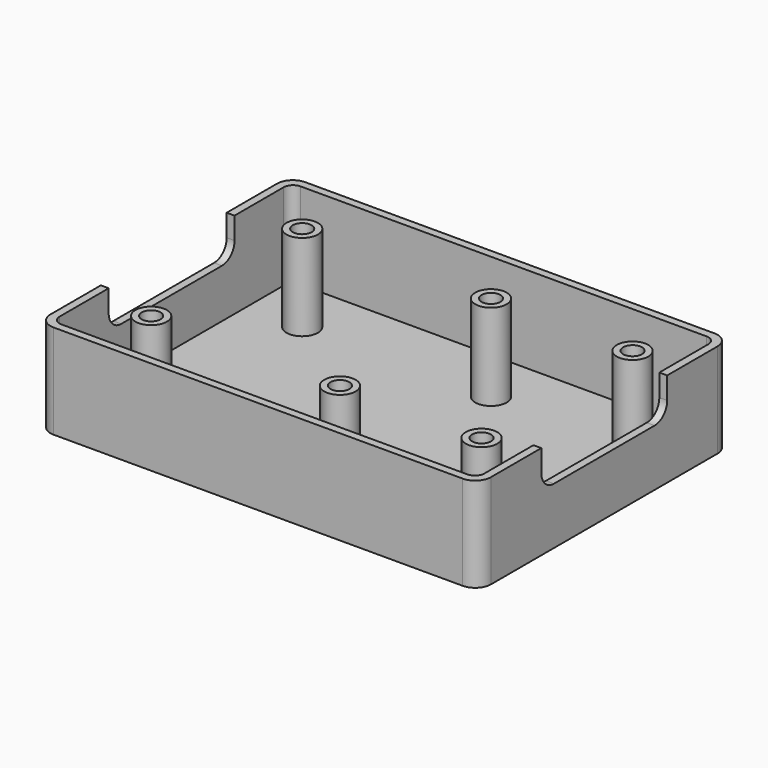
from build123d import *

# Parameters (mm, degrees)
F0_W          = 140
F0_H          = 100
F1_DEPTH      = 30
F2_T          = -2.5
F3_W          = 50
F3_H          = 12
F4_DEPTH      = 205.5
F5_R          = 5
F6_R          = 5
F7_R          = 3
F8_R          = 5
F9_DEPTH      = 27.5
F10_T         = 2
F10_T3_DEPTH  = 93
F10_T5_DEPTH  = 133
F10_T8_ANGLE  = 90.000000001
F10_T10_ANGLE = 90.000000001
F10_T12_ANGLE = 90.000000001
F10_T14_ANGLE = 90.000000001
F11_ANGLE     = 60
F12_ANGLE     = 30
F13_ANGLE     = 90


# Not quite as in the source:
# - a shell that OpenCascade refuses in one call is made with other operations: the cavity is built on its own and cut out


with BuildPart() as f1:
    # F0 (on Top) → F1 (new body)
    with BuildSketch(Plane.XY):
        with Locations((50, 0)):
            Rectangle(F0_W, F0_H)
    extrude(amount=F1_DEPTH)

    # F2
    f2_openings = [f1.faces().sort_by_distance(p)[0] for p in [
        (50, 0, 30),
    ]]
    offset(amount=F2_T, openings=f2_openings)

    # F3 (on face) → F4 (cut)
    with BuildSketch(Plane.YZ.offset(120)):
        with Locations((0, 24)):
            Rectangle(F3_W, F3_H)
    extrude(amount=-F4_DEPTH, mode=Mode.SUBTRACT)

    # F5
    f5_edges = [f1.edges().sort_by_distance(p)[0] for p in [
        (-18.75, 25, 18),
        (-18.75, -25, 18),
        (118.75, -25, 18),
        (118.75, 25, 18),
    ]]
    fillet(f5_edges, radius=F5_R)

    # F6
    f6_edges = [f1.edges().sort_by_distance(p)[0] for p in [
        (120, 50, 15),
        (-20, 50, 15),
        (-20, -50, 15),
        (120, -50, 15),
    ]]
    fillet(f6_edges, radius=F6_R)

    # F7
    f7_edges = [f1.edges().sort_by_distance(p)[0] for p in [
        (-17.5, -47.5, 16.25),
        (-17.5, 47.5, 16.25),
        (117.5, 47.5, 16.25),
        (117.5, -47.5, 16.25),
    ]]
    fillet(f7_edges, radius=F7_R)

    # F8 (on face) → F9 (join, through all)
    with BuildSketch(Plane.XY.offset(2.5)):
        with Locations((-5, -30)):
            Circle(F8_R)
        with Locations((40, -30)):
            Circle(F8_R)
        with Locations((100, -30)):
            Circle(F8_R)
        with Locations((100, 30)):
            Circle(F8_R)
        with Locations((40, 30)):
            Circle(F8_R)
        with Locations((-5, 30)):
            Circle(F8_R)
    extrude(amount=F9_DEPTH)

    # F10: shell of thickness 2, made by hand


with BuildPart() as f10_core1:
    # F10_t2: copy of F1
    add(f1.part)

    # the walls: a layer under each face that stays
    f10_faces = [f10_core1.faces().sort_by_distance(p)[0] for p in [
        (-10, -48.2142857143, 30),
        (117.5, 0, 16.25),
        (116.6213203436, -46.6213203436, 16.25),
        (118.75, -25, 26.5),
        (50, -47.5, 16.25),
        (120, 0, 15),
        (-16.6213203436, -46.6213203436, 16.25),
        (118.5355339059, -48.5355339059, 15),
        (-17.5, 0, 16.25),
        (50, -50, 15),
        (-18.75, -25, 26.5),
        (-18.5355339059, -48.5355339059, 15),
        (-20, 0, 15),
        (-10, 48.2142857143, 30),
        (116.6213203436, 46.6213203436, 16.25),
        (118.75, 25, 26.5),
        (50, 0, 2.5),
        (118.75, 23.5355339059, 19.4644660941),
        (118.75, 0, 18),
        (118.75, -23.5355339059, 19.4644660941),
        (118.5355339059, 48.5355339059, 15),
        (50, 0, 0),
        (-18.75, -23.5355339059, 19.4644660941),
        (-16.6213203436, 46.6213203436, 16.25),
        (-18.75, 0, 18),
        (-18.75, 23.5355339059, 19.4644660941),
        (-18.75, 25, 26.5),
        (-18.5355339059, 48.5355339059, 15),
        (50, 47.5, 16.25),
        (50, 50, 15),
        (-10, -30, 16.25),
        (35, -30, 16.25),
        (95, -30, 16.25),
        (-10, 30, 16.25),
        (35, 30, 16.25),
        (95, 30, 16.25),
    ]]
    thicken(f10_faces, amount=-F10_T, mode=Mode.SUBTRACT)

    # F10_s4 → F10_t3 (cut)
    with BuildSketch(Plane.XZ.offset(-46.5)):
        Polygon((117.48, 2.52), (119.5, 2.5), (119.5, 0.5), (117.5, 0.5), align=None)
        Polygon((-17.48, 2.52), (-19.5, 2.5), (-19.5, 0.5), (-17.5, 0.5), align=None)
    extrude(amount=F10_T3_DEPTH, mode=Mode.SUBTRACT)

    # F10_s6 → F10_t5 (cut)
    with BuildSketch(Plane.YZ.offset(-16.5)):
        Polygon((-47.48, 2.52), (-49.5, 2.5), (-49.5, 0.5), (-47.5, 0.5), align=None)
        Polygon((47.48, 2.52), (47.5, 0.5), (49.5, 0.5), (49.5, 2.5), align=None)
    extrude(amount=F10_T5_DEPTH, mode=Mode.SUBTRACT)

    # F10_s7 → F10_t8 (revolve, cut)
    with BuildSketch(Plane.XZ.offset(44.5)):
        Polygon((117.48, 2.52), (119.5, 2.5), (119.5, 0.5), (117.5, 0.5), align=None)
    revolve(axis=Axis((114.5, -44.5, 2.5), (0, 0, -1)), revolution_arc=F10_T8_ANGLE, mode=Mode.SUBTRACT)

    # F10_s9 → F10_t10 (revolve, cut)
    with BuildSketch(Plane.YZ.offset(-14.5)):
        Polygon((-47.48, 2.52), (-49.5, 2.5), (-49.5, 0.5), (-47.5, 0.5), align=None)
    revolve(axis=Axis((-14.5, -44.5, 2.5), (0, 0, -1)), revolution_arc=F10_T10_ANGLE, mode=Mode.SUBTRACT)

    # F10_s11 → F10_t12 (revolve, cut)
    with BuildSketch(Plane.XZ.offset(-44.5)):
        Polygon((117.48, 2.52), (119.5, 2.5), (119.5, 0.5), (117.5, 0.5), align=None)
    revolve(axis=Axis((114.5, 44.5, 2.5), (0, 0, 1)), revolution_arc=F10_T12_ANGLE, mode=Mode.SUBTRACT)

    # F10_s13 → F10_t14 (revolve, cut)
    with BuildSketch(Plane.XZ.offset(-44.5)):
        Polygon((-17.48, 2.52), (-17.5, 0.5), (-19.5, 0.5), (-19.5, 2.5), align=None)
    revolve(axis=Axis((-14.5, 44.5, 2.5), (0, 0, -1)), revolution_arc=F10_T14_ANGLE, mode=Mode.SUBTRACT)

    # F10_s15 → F10_t16 (revolve, cut)
    with BuildSketch(Plane.XZ.offset(30)):
        Polygon((0.02, 2.52), (0, 0.5), (-2, 0.5), (-2, 2.5), align=None)
    revolve(axis=Axis((-5, -30, 2.5), (0, 0, 1)), mode=Mode.SUBTRACT)

    # F10_s17 → F10_t18 (revolve, cut)
    with BuildSketch(Plane.XZ.offset(30)):
        Polygon((45.02, 2.52), (45, 0.5), (43, 0.5), (43, 2.5), align=None)
    revolve(axis=Axis((40, -30, 2.5), (0, 0, 1)), mode=Mode.SUBTRACT)

    # F10_s19 → F10_t20 (revolve, cut)
    with BuildSketch(Plane.XZ.offset(30)):
        Polygon((105.02, 2.52), (105, 0.5), (103, 0.5), (103, 2.5), align=None)
    revolve(axis=Axis((100, -30, 2.5), (0, 0, 1)), mode=Mode.SUBTRACT)

    # F10_s21 → F10_t22 (revolve, cut)
    with BuildSketch(Plane.XZ.offset(-30)):
        Polygon((0.02, 2.52), (0, 0.5), (-2, 0.5), (-2, 2.5), align=None)
    revolve(axis=Axis((-5, 30, 2.5), (0, 0, 1)), mode=Mode.SUBTRACT)

    # F10_s23 → F10_t24 (revolve, cut)
    with BuildSketch(Plane.XZ.offset(-30)):
        Polygon((45.02, 2.52), (45, 0.5), (43, 0.5), (43, 2.5), align=None)
    revolve(axis=Axis((40, 30, 2.5), (0, 0, 1)), mode=Mode.SUBTRACT)

    # F10_s25 → F10_t26 (revolve, cut)
    with BuildSketch(Plane.XZ.offset(-30)):
        Polygon((105.02, 2.52), (105, 0.5), (103, 0.5), (103, 2.5), align=None)
    revolve(axis=Axis((100, 30, 2.5), (0, 0, 1)), mode=Mode.SUBTRACT)


with BuildPart() as f1_1:
    add(f1.part)

    # what is left inside the walls is the cavity
    f10_cavity = [f10_core1.part.solids().sort_by_distance(p)[0] for p in [
        (-7.98, -30, 11.333333),
        (37.02, -30, 11.333333),
        (97.02, -30, 11.333333),
        (-7.98, 30, 11.333333),
        (37.02, 30, 11.333333),
        (97.02, 30, 11.333333),
    ]]
    add(f10_cavity, mode=Mode.SUBTRACT)


with BuildPart() as f1_2:
    # F11: moved
    add(f1_1.part.rotate(Axis((-5, 30, 2), (0, 0, 1)), F11_ANGLE))


with BuildPart() as f1_3:
    # F12: moved
    add(f1_2.part.rotate(Axis((47.5, 120.9326673974, 0.5), (0, 0, 1)), F12_ANGLE))


with BuildPart() as f1_4:
    # F13: moved
    add(f1_3.part.rotate(Axis((47.5, 120.9326673974, 0.5), (0, 0, 1)), F13_ANGLE))


solid = f1_4.part
